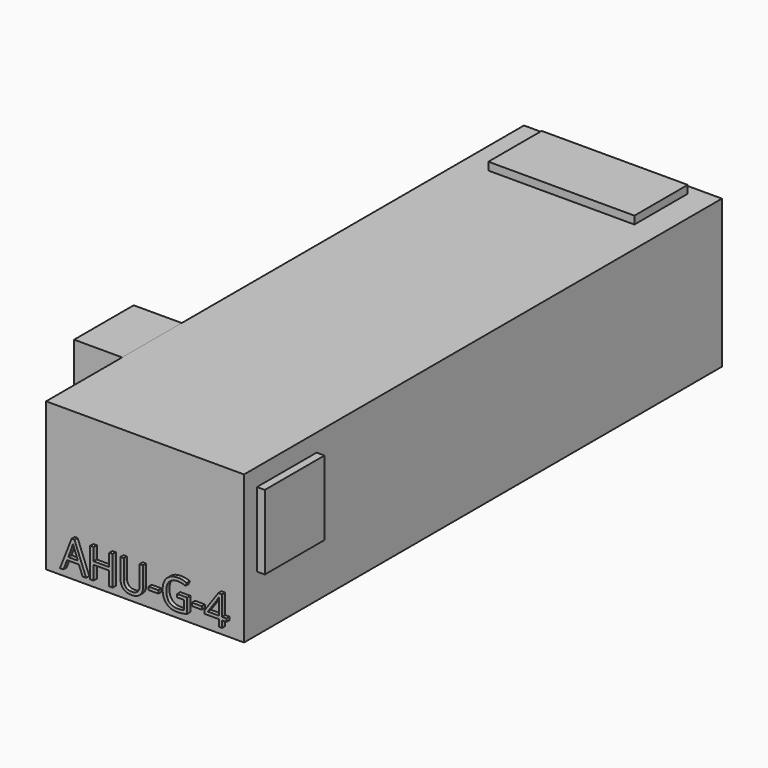
from build123d import *

# Parameters (mm, degrees)
F0_W         = 1282.7
F0_H         = 958.85
F1_DEPTH     = 3870.325
F2_W         = 482.6
F2_H         = 482.6
F3_DEPTH     = 50.8
F4_W         = 482.6
F4_H         = 762
F5_DEPTH     = 311.15
F6_TEXT_SIZE = 268.1662225061
F7_DEPTH     = 25.4
F8_W         = 946.15
F8_H         = 431.8
F9_DEPTH     = 50.8
F10_W        = 946.15
F10_H        = 431.8
F11_DEPTH    = 50.8


# Not quite as in the source:
# - Text() gives the source's letters only with a copy of the font that has no kerning and outlines rounded to 1/6400 em; it was checked with that copy


with BuildPart() as f1:
    # F0 (on Front) → F1 (new body)
    with BuildSketch(Plane.XZ):
        with Locations((1.4098696411, -73.0132179465)):
            Rectangle(F0_W, F0_H)
    extrude(amount=F1_DEPTH)

    # F2 (on face) → F3 (join)
    with BuildSketch(Plane.YZ.offset(642.7598696411)):
        with Locations((-3524.25, 50.8117820535)):
            Rectangle(F2_W, F2_H)
    extrude(amount=F3_DEPTH)

    # F6 (on face) → F7 (join)
    with BuildSketch(Plane.XZ.offset(3870.325)):
        with Locations((-529.784437269, -499.1856813431)):
            Text('AHU-G-4', F6_TEXT_SIZE, font='Open Sans', text_align=(TextAlign.LEFT, TextAlign.BOTTOM))
    extrude(amount=F7_DEPTH)

    # F8 (on face) → F9 (join)
    with BuildSketch(Plane.XY.offset(406.4117820535)):
        with Locations((1.4098696411, -282.575)):
            Rectangle(F8_W, F8_H)
    extrude(amount=F9_DEPTH)

    # F10 (on face) → F11 (join)
    with BuildSketch(Plane(origin=(0, 0, 0), x_dir=(-1, 0, 0), z_dir=(0, 1, 0))):
        with Locations((-1.4098696411, -38.0882179465)):
            Rectangle(F10_W, F10_H)
    extrude(amount=F11_DEPTH)


with BuildPart() as f5:
    # F4 (on face) → F5 (new body)
    with BuildSketch(Plane(origin=(-639.9401303589, 0, 0), x_dir=(0, -1, 0), z_dir=(-1, 0, 0))):
        with Locations((3013.075, 25.4117820535)):
            Rectangle(F4_W, F4_H)
    extrude(amount=F5_DEPTH)


solid = Compound([f1.part, f5.part])
